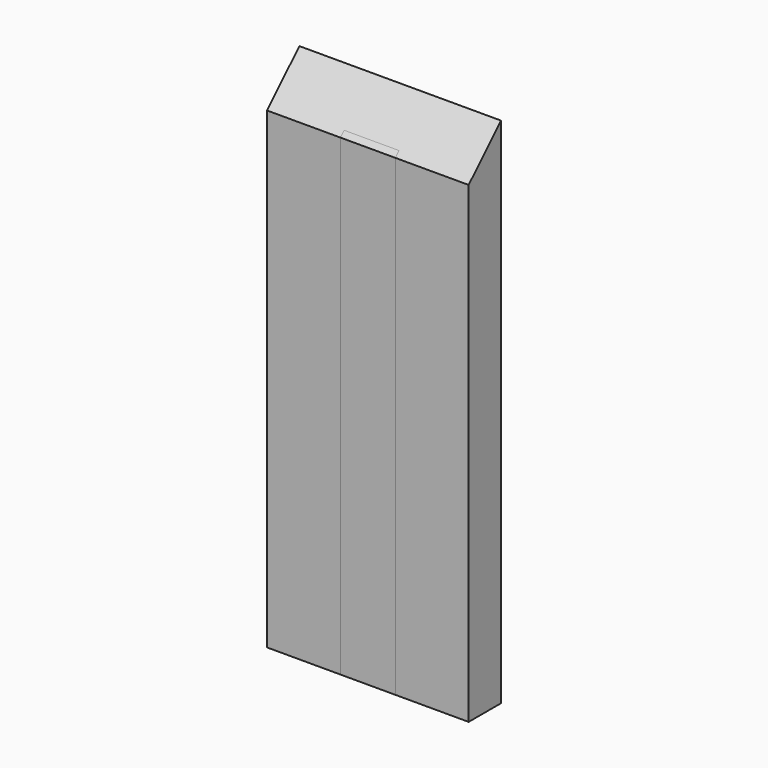
from build123d import *

# Parameters (mm, degrees)
F0_W     = 139.7
F0_H     = 27.94
F1_DEPTH = 355.6
F2_SIZE  = 27.93999
F3_W     = 38.1
F3_H     = 355.6
F4_DEPTH = 3.175
F5_DEPTH = 38.1


# Not quite as in the source:
# - a fillet or chamfer is up to 0.001 mm smaller than in the source, because OpenCascade refuses the exact size


with BuildPart() as f1:
    # F0 (on Top) → F1 (new body)
    with BuildSketch(Plane.XY):
        with Locations((69.85, -13.97)):
            Rectangle(F0_W, F0_H)
    extrude(amount=F1_DEPTH)

    # F2 (size 27.94 in the source; OpenCascade refuses exactly that, so slightly less here)
    f2_edges = [f1.edges().sort_by_distance(p)[0] for p in [
        (69.85, -27.94, 355.6),
    ]]
    chamfer(f2_edges, length=F2_SIZE)

    # F3 (on face) → F4 (cut)
    with BuildSketch(Plane.XZ.offset(27.94)):
        with Locations((69.85, 177.8)):
            Rectangle(F3_W, F3_H)
    extrude(amount=-F4_DEPTH, mode=Mode.SUBTRACT)


with BuildPart() as f5:
    # F5 (new, through all): a face of the model
    f5_faces = [f1.part.faces().sort_by_distance(p)[0] for p in [
        (50.8, -26.3499485697, 164.6250307152),
    ]]
    extrude(f5_faces, amount=F5_DEPTH)


solid = Compound([f1.part, f5.part])
